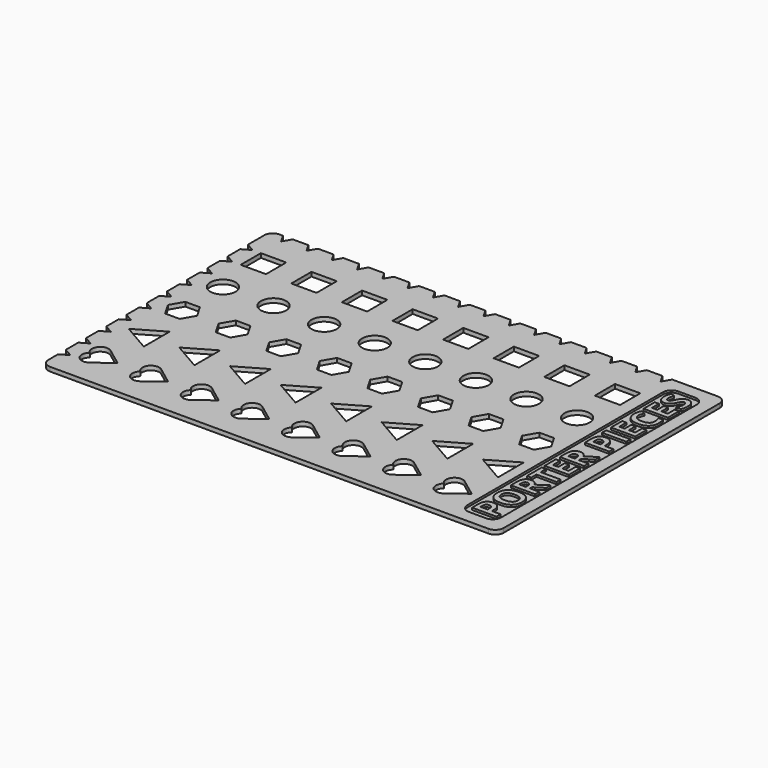
from build123d import *

# Parameters (mm, degrees)
F0_W          = 85.725
F0_H          = 53.975
F1_DEPTH      = 0.79375
F2_R          = 1.5875
F3_W          = 4.7625
F3_H          = 4.7625
F4_DEPTH      = 25.4
F6_DEPTH      = 25.4
F8_DEPTH      = 25.4
F9_R          = 2.38125
F10_DEPTH     = 25.4
F12_DEPTH     = 25.4
F14_DEPTH     = 25.4
F16_DEPTH     = 25.4
F18_DEPTH     = 25.4
F19_W         = 6.35
F19_H         = 49.2125
F20_DEPTH     = 0.396875
F21_R         = 1.5875
F22_TEXT_SIZE = 6.4051106395
F23_DEPTH     = 0.396875
F25_DEPTH     = 25.4
F27_DEPTH     = 25.4


# Not quite as in the source:
# - a feature names something its author has since deleted; it is built from what else it names
# - Text() gives the source's letters only with a copy of the font that has no kerning and outlines rounded to 1/6400 em; it was checked with that copy


with BuildPart() as f1:
    # F0 (on Top) → F1 (new body)
    with BuildSketch(Plane.XY):
        Rectangle(F0_W, F0_H)
    extrude(amount=F1_DEPTH)

    # F2
    f2_edges = [f1.edges().sort_by_distance(p)[0] for p in [
        (42.8625, 26.9875, 0.396875),
        (-42.8625, 26.9875, 0.396875),
        (-42.8625, -26.9875, 0.396875),
        (42.8625, -26.9875, 0.396875),
    ]]
    fillet(f2_edges, radius=F2_R)

    # F3 (on face) → F4 (cut)
    with BuildSketch(Plane.XY.offset(0.79375)):
        with Locations((-37.30625, 18.25625)):
            Rectangle(F3_W, F3_H)
        with Locations((-27.78125, 18.25625)):
            Rectangle(F3_W, F3_H)
        with Locations((-18.25625, 18.25625)):
            Rectangle(F3_W, F3_H)
        with Locations((-8.73125, 18.25625)):
            Rectangle(F3_W, F3_H)
        with Locations((0.79375, 18.25625)):
            Rectangle(F3_W, F3_H)
        with Locations((10.31875, 18.25625)):
            Rectangle(F3_W, F3_H)
        with Locations((19.84375, 18.25625)):
            Rectangle(F3_W, F3_H)
        with Locations((29.36875, 18.25625)):
            Rectangle(F3_W, F3_H)
    extrude(amount=-F4_DEPTH, mode=Mode.SUBTRACT)

    # F5 (on face) → F6 (cut)
    with BuildSketch(Plane.XY.offset(0.79375)):
        Polygon((-34.0084564477, 26.9875), (-35.8415435523, 26.9875), (-34.925, 25.4), align=None)
        Polygon((-29.2459564477, 26.9875), (-31.0790435523, 26.9875), (-30.1625, 25.4), align=None)
        Polygon((-24.4834564477, 26.9875), (-26.3165435523, 26.9875), (-25.4, 25.4), align=None)
        Polygon((-19.7209564477, 26.9875), (-21.5540435523, 26.9875), (-20.6375, 25.4), align=None)
        Polygon((-14.9584564477, 26.9875), (-16.7915435523, 26.9875), (-15.875, 25.4), align=None)
        Polygon((-10.1959564477, 26.9875), (-12.0290435523, 26.9875), (-11.1125, 25.4), align=None)
        Polygon((-5.4334564477, 26.9875), (-7.2665435523, 26.9875), (-6.35, 25.4), align=None)
        Polygon((-0.6709564477, 26.9875), (-2.5040435523, 26.9875), (-1.5875, 25.4), align=None)
        Polygon((8.8540435523, 26.9875), (7.0209564477, 26.9875), (7.9375, 25.4), align=None)
        Polygon((4.0915435523, 26.9875), (2.2584564477, 26.9875), (3.175, 25.4), align=None)
        Polygon((12.7, 25.4), (13.6165435523, 26.9875), (11.7834564477, 26.9875), align=None)
        Polygon((17.4625, 25.4), (18.3790435523, 26.9875), (16.5459564477, 26.9875), align=None)
        Polygon((31.75, 25.4), (32.6665435523, 26.9875), (30.8334564477, 26.9875), align=None)
        Polygon((26.9875, 25.4), (27.9040435523, 26.9875), (26.0709564477, 26.9875), align=None)
        Polygon((22.225, 25.4), (23.1415435523, 26.9875), (21.3084564477, 26.9875), align=None)
    extrude(amount=-F6_DEPTH, mode=Mode.SUBTRACT)

    # F7 (on face) → F8 (cut)
    with BuildSketch(Plane.XY.offset(0.79375)):
        Polygon((-38.7709564477, 26.9875), (-40.6040435523, 26.9875), (-39.6875, 25.4), align=None)
    extrude(amount=-F8_DEPTH, mode=Mode.SUBTRACT)

    # F9 (on face) → F10 (cut)
    with BuildSketch(Plane.XY.offset(0.79375)):
        with Locations((-37.30625, 8.73125)):
            Circle(F9_R)
        with Locations((-27.78125, 8.73125)):
            Circle(F9_R)
        with Locations((-18.25625, 8.73125)):
            Circle(F9_R)
        with Locations((-8.73125, 8.73125)):
            Circle(F9_R)
        with Locations((0.79375, 8.73125)):
            Circle(F9_R)
        with Locations((10.31875, 8.73125)):
            Circle(F9_R)
        with Locations((19.84375, 8.73125)):
            Circle(F9_R)
        with Locations((29.36875, 8.73125)):
            Circle(F9_R)
    extrude(amount=-F10_DEPTH, mode=Mode.SUBTRACT)

    # F11 (on face) → F12 (cut)
    with BuildSketch(Plane.XY.offset(0.79375)):
        Polygon((-35.9314346715, 1.5875), (-38.6810653285, 1.5875), (-40.055880657, -0.79375), (-38.6810653285, -3.175), (-35.9314346715, -3.175), (-34.556619343, -0.79375), align=None)
        Polygon((-26.4064346715, 1.5875), (-29.1560653285, 1.5875), (-30.530880657, -0.79375), (-29.1560653285, -3.175), (-26.4064346715, -3.175), (-25.031619343, -0.79375), align=None)
        Polygon((-16.8814346715, 1.5875), (-19.6310653285, 1.5875), (-21.005880657, -0.79375), (-19.6310653285, -3.175), (-16.8814346715, -3.175), (-15.506619343, -0.79375), align=None)
        Polygon((-7.3564346715, 1.5875), (-10.1060653285, 1.5875), (-11.480880657, -0.79375), (-10.1060653285, -3.175), (-7.3564346715, -3.175), (-5.981619343, -0.79375), align=None)
        Polygon((2.1685653285, 1.5875), (-0.5810653285, 1.5875), (-1.955880657, -0.79375), (-0.5810653285, -3.175), (2.1685653285, -3.175), (3.543380657, -0.79375), align=None)
        Polygon((11.6935653285, 1.5875), (8.9439346715, 1.5875), (7.569119343, -0.79375), (8.9439346715, -3.175), (11.6935653285, -3.175), (13.068380657, -0.79375), align=None)
        Polygon((21.2185653285, 1.5875), (18.4689346715, 1.5875), (17.094119343, -0.79375), (18.4689346715, -3.175), (21.2185653285, -3.175), (22.593380657, -0.79375), align=None)
        Polygon((30.7435653285, 1.5875), (27.9939346715, 1.5875), (26.619119343, -0.79375), (27.9939346715, -3.175), (30.7435653285, -3.175), (32.118380657, -0.79375), align=None)
    extrude(amount=-F12_DEPTH, mode=Mode.SUBTRACT)

    # F13 (on face) → F14 (cut)
    with BuildSketch(Plane.XY.offset(0.79375)):
        Polygon((-34.925, -12.7), (-34.925, -7.9375), (-39.0494459855, -10.31875), align=None)
        Polygon((-25.4, -7.9375), (-29.5244459855, -10.31875), (-25.4, -12.7), align=None)
        Polygon((-15.875, -7.9375), (-19.9994459855, -10.31875), (-15.875, -12.7), align=None)
        Polygon((-6.35, -7.9375), (-10.4744459855, -10.31875), (-6.35, -12.7), align=None)
        Polygon((3.175, -7.9375), (-0.9494459855, -10.31875), (3.175, -12.7), align=None)
        Polygon((12.7, -7.9375), (8.5755540145, -10.31875), (12.7, -12.7), align=None)
        Polygon((22.225, -7.9375), (18.1005540145, -10.31875), (22.225, -12.7), align=None)
        Polygon((31.75, -7.9375), (27.6255540145, -10.31875), (31.75, -12.7), align=None)
    extrude(amount=-F14_DEPTH, mode=Mode.SUBTRACT)

    # F15 (on face) → F16 (cut)
    with BuildSketch(Plane.XY.offset(0.79375)):
        with BuildLine():
            ThreePointArc((-37.7825, -17.700625), (-39.6264010517, -18.2766163161), (-38.496875, -19.84375))
            ThreePointArc((-38.496875, -19.84375), (-39.6264010517, -21.4108836839), (-37.7825, -21.986875))
            Line((-37.7825, -21.986875), (-34.925, -19.84375))
            Line((-34.925, -19.84375), (-37.7825, -17.700625))
        make_face()
        with BuildLine():
            ThreePointArc((-28.2575, -17.700625), (-30.1014010517, -18.2766163161), (-28.971875, -19.84375))
            ThreePointArc((-28.971875, -19.84375), (-30.1014010517, -21.4108836839), (-28.2575, -21.986875))
            Line((-28.2575, -21.986875), (-25.4, -19.84375))
            Line((-25.4, -19.84375), (-28.2575, -17.700625))
        make_face()
        with BuildLine():
            ThreePointArc((-18.7325, -17.700625), (-20.5764010517, -18.2766163161), (-19.446875, -19.84375))
            ThreePointArc((-19.446875, -19.84375), (-20.5764010517, -21.4108836839), (-18.7325, -21.986875))
            Line((-18.7325, -21.986875), (-15.875, -19.84375))
            Line((-15.875, -19.84375), (-18.7325, -17.700625))
        make_face()
        with BuildLine():
            ThreePointArc((-9.2075, -17.700625), (-11.0514010517, -18.2766163161), (-9.921875, -19.84375))
            ThreePointArc((-9.921875, -19.84375), (-11.0514010517, -21.4108836839), (-9.2075, -21.986875))
            Line((-9.2075, -21.986875), (-6.35, -19.84375))
            Line((-6.35, -19.84375), (-9.2075, -17.700625))
        make_face()
        with BuildLine():
            ThreePointArc((0.3175, -17.700625), (-1.5264010517, -18.2766163161), (-0.396875, -19.84375))
            ThreePointArc((-0.396875, -19.84375), (-1.5264010517, -21.4108836839), (0.3175, -21.986875))
            Line((0.3175, -21.986875), (3.175, -19.84375))
            Line((3.175, -19.84375), (0.3175, -17.700625))
        make_face()
        with BuildLine():
            ThreePointArc((9.8425, -17.700625), (7.9985989483, -18.2766163161), (9.128125, -19.84375))
            ThreePointArc((9.128125, -19.84375), (7.9985989483, -21.4108836839), (9.8425, -21.986875))
            Line((9.8425, -21.986875), (12.7, -19.84375))
            Line((12.7, -19.84375), (9.8425, -17.700625))
        make_face()
        with BuildLine():
            ThreePointArc((19.3675, -17.700625), (17.5235989483, -18.2766163161), (18.653125, -19.84375))
            ThreePointArc((18.653125, -19.84375), (17.5235989483, -21.4108836839), (19.3675, -21.986875))
            Line((19.3675, -21.986875), (22.225, -19.84375))
            Line((22.225, -19.84375), (19.3675, -17.700625))
        make_face()
        with BuildLine():
            ThreePointArc((28.8925, -17.700625), (27.0485989483, -18.2766163161), (28.178125, -19.84375))
            ThreePointArc((28.178125, -19.84375), (27.0485989483, -21.4108836839), (28.8925, -21.986875))
            Line((28.8925, -21.986875), (31.75, -19.84375))
            Line((31.75, -19.84375), (28.8925, -17.700625))
        make_face()
    extrude(amount=-F16_DEPTH, mode=Mode.SUBTRACT)

    # F17 (on face) → F18 (cut)
    with BuildSketch(Plane(origin=(0, 0, 0), x_dir=(1, 0, 0), z_dir=(0, 0, -1))):
        Polygon((-42.8625, -19.7209564477), (-42.8625, -21.5540435523), (-41.275, -20.6375), align=None)
        Polygon((-42.8625, -14.9584564477), (-42.8625, -16.7915435523), (-41.275, -15.875), align=None)
        Polygon((-42.8625, -10.1959564477), (-42.8625, -12.0290435523), (-41.275, -11.1125), align=None)
        Polygon((-42.8625, -5.4334564477), (-42.8625, -7.2665435523), (-41.275, -6.35), align=None)
        Polygon((-42.8625, -0.6709564477), (-42.8625, -2.5040435523), (-41.275, -1.5875), align=None)
        Polygon((-42.8625, 4.0915435523), (-42.8625, 2.2584564477), (-41.275, 3.175), align=None)
        Polygon((-42.8625, 8.8540435523), (-42.8625, 7.0209564477), (-41.275, 7.9375), align=None)
        Polygon((-42.8625, 13.6165435523), (-42.8625, 11.7834564477), (-41.275, 12.7), align=None)
        Polygon((-42.8625, 18.3790435523), (-42.8625, 16.5459564477), (-41.275, 17.4625), align=None)
        Polygon((-42.8625, 23.1415435523), (-42.8625, 21.3084564477), (-41.275, 22.225), align=None)
    extrude(amount=-F18_DEPTH, mode=Mode.SUBTRACT)

    # F19 (on face) → F20 (cut)
    with BuildSketch(Plane.XY.offset(0.79375)):
        with Locations((37.30625, 0)):
            Rectangle(F19_W, F19_H)
    extrude(amount=-F20_DEPTH, mode=Mode.SUBTRACT)

    # F21
    f21_edges = [f1.edges().sort_by_distance(p)[0] for p in [
        (34.13125, -24.60625, 0.595313),
        (40.48125, -24.60625, 0.595313),
        (40.48125, 24.60625, 0.595313),
        (34.13125, 24.60625, 0.595313),
    ]]
    fillet(f21_edges, radius=F21_R)

    # F22 (on face) → F23 (join)
    with BuildSketch(Plane.XY.offset(0.396875)):
        with Locations(Location((39.7566241945, -23.8125), (0, 0, 90))):
            Text('PORTER PIECES', F22_TEXT_SIZE, font='Open Sans', font_style=FontStyle.BOLD, text_align=(TextAlign.LEFT, TextAlign.BOTTOM))
    extrude(amount=F23_DEPTH)

    # F24 (on face) → F25 (cut)
    with BuildSketch(Plane.XY.offset(0.79375)):
        Polygon((-39.8114459855, -10.31875), (-34.544, -13.3599113577), (-34.544, -7.2775886423), align=None)
        Polygon((-34.925, -7.9375), (-34.925, -12.7), (-39.0494459855, -10.31875), align=None, mode=Mode.SUBTRACT)
        Polygon((-25.019, -13.3599113577), (-25.019, -7.2775886423), (-30.2864459855, -10.31875), align=None)
        Polygon((-25.4, -12.7), (-29.5244459855, -10.31875), (-25.4, -7.9375), align=None, mode=Mode.SUBTRACT)
        Polygon((-15.494, -13.3599113577), (-15.494, -7.2775886423), (-20.7614459855, -10.31875), align=None)
        Polygon((-15.875, -12.7), (-19.9994459855, -10.31875), (-15.875, -7.9375), align=None, mode=Mode.SUBTRACT)
        Polygon((-5.969, -13.3599113577), (-5.969, -7.2775886423), (-11.2364459855, -10.31875), align=None)
        Polygon((-6.35, -12.7), (-10.4744459855, -10.31875), (-6.35, -7.9375), align=None, mode=Mode.SUBTRACT)
        Polygon((3.556, -13.3599113577), (3.556, -7.2775886423), (-1.7114459855, -10.31875), align=None)
        Polygon((3.175, -12.7), (-0.9494459855, -10.31875), (3.175, -7.9375), align=None, mode=Mode.SUBTRACT)
        Polygon((13.081, -13.3599113577), (13.081, -7.2775886423), (7.8135540145, -10.31875), align=None)
        Polygon((12.7, -12.7), (8.5755540145, -10.31875), (12.7, -7.9375), align=None, mode=Mode.SUBTRACT)
        Polygon((22.606, -13.3599113577), (22.606, -7.2775886423), (17.3385540145, -10.31875), align=None)
        Polygon((22.225, -12.7), (18.1005540145, -10.31875), (22.225, -7.9375), align=None, mode=Mode.SUBTRACT)
        Polygon((32.131, -13.3599113577), (32.131, -7.2775886423), (26.8635540145, -10.31875), align=None)
        Polygon((31.75, -12.7), (27.6255540145, -10.31875), (31.75, -7.9375), align=None, mode=Mode.SUBTRACT)
    extrude(amount=-F25_DEPTH, mode=Mode.SUBTRACT)

    # F26 (on face) → F27 (cut)
    with BuildSketch(Plane.XY.offset(0.79375)):
        with BuildLine():
            Line((-37.5539, -22.291675), (-34.29, -19.84375))
            Line((-34.29, -19.84375), (-37.5539, -17.395825))
            ThreePointArc((-37.5539, -17.395825), (-39.721539141, -17.6681362272), (-39.5227488958, -19.84375))
            ThreePointArc((-39.5227488958, -19.84375), (-39.721539141, -22.0193637728), (-37.5539, -22.291675))
        make_face()
        with BuildLine():
            ThreePointArc((-37.7825, -21.986875), (-39.6264010517, -21.4108836839), (-38.496875, -19.84375))
            ThreePointArc((-38.496875, -19.84375), (-39.6264010517, -18.2766163161), (-37.7825, -17.700625))
            Line((-37.7825, -17.700625), (-34.925, -19.84375))
            Line((-34.925, -19.84375), (-37.7825, -21.986875))
        make_face(mode=Mode.SUBTRACT)
        with BuildLine():
            Line((-28.0289, -22.291675), (-24.765, -19.84375))
            Line((-24.765, -19.84375), (-28.0289, -17.395825))
            ThreePointArc((-28.0289, -17.395825), (-30.196539141, -17.6681362272), (-29.9977488958, -19.84375))
            ThreePointArc((-29.9977488958, -19.84375), (-30.196539141, -22.0193637728), (-28.0289, -22.291675))
        make_face()
        with BuildLine():
            ThreePointArc((-28.971875, -19.84375), (-30.1014010517, -18.2766163161), (-28.2575, -17.700625))
            Line((-28.2575, -17.700625), (-25.4, -19.84375))
            Line((-25.4, -19.84375), (-28.2575, -21.986875))
            ThreePointArc((-28.2575, -21.986875), (-30.1014010517, -21.4108836839), (-28.971875, -19.84375))
        make_face(mode=Mode.SUBTRACT)
        with BuildLine():
            Line((-18.5039, -22.291675), (-15.24, -19.84375))
            Line((-15.24, -19.84375), (-18.5039, -17.395825))
            ThreePointArc((-18.5039, -17.395825), (-20.671539141, -17.6681362272), (-20.4727488958, -19.84375))
            ThreePointArc((-20.4727488958, -19.84375), (-20.671539141, -22.0193637728), (-18.5039, -22.291675))
        make_face()
        with BuildLine():
            Line((-18.7325, -17.700625), (-15.875, -19.84375))
            Line((-15.875, -19.84375), (-18.7325, -21.986875))
            ThreePointArc((-18.7325, -21.986875), (-20.5764010517, -21.4108836839), (-19.446875, -19.84375))
            ThreePointArc((-19.446875, -19.84375), (-20.5764010517, -18.2766163161), (-18.7325, -17.700625))
        make_face(mode=Mode.SUBTRACT)
        with BuildLine():
            Line((-8.9789, -22.291675), (-5.715, -19.84375))
            Line((-5.715, -19.84375), (-8.9789, -17.395825))
            ThreePointArc((-8.9789, -17.395825), (-11.146539141, -17.6681362272), (-10.9477488958, -19.84375))
            ThreePointArc((-10.9477488958, -19.84375), (-11.146539141, -22.0193637728), (-8.9789, -22.291675))
        make_face()
        with BuildLine():
            ThreePointArc((-9.921875, -19.84375), (-11.0514010517, -18.2766163161), (-9.2075, -17.700625))
            Line((-9.2075, -17.700625), (-6.35, -19.84375))
            Line((-6.35, -19.84375), (-9.2075, -21.986875))
            ThreePointArc((-9.2075, -21.986875), (-11.0514010517, -21.4108836839), (-9.921875, -19.84375))
        make_face(mode=Mode.SUBTRACT)
        with BuildLine():
            Line((0.5461, -22.291675), (3.81, -19.84375))
            Line((3.81, -19.84375), (0.5461, -17.395825))
            ThreePointArc((0.5461, -17.395825), (-1.621539141, -17.6681362272), (-1.4227488958, -19.84375))
            ThreePointArc((-1.4227488958, -19.84375), (-1.621539141, -22.0193637728), (0.5461, -22.291675))
        make_face()
        with BuildLine():
            Line((0.3175, -17.700625), (3.175, -19.84375))
            Line((3.175, -19.84375), (0.3175, -21.986875))
            ThreePointArc((0.3175, -21.986875), (-1.5264010517, -21.4108836839), (-0.396875, -19.84375))
            ThreePointArc((-0.396875, -19.84375), (-1.5264010517, -18.2766163161), (0.3175, -17.700625))
        make_face(mode=Mode.SUBTRACT)
        with BuildLine():
            Line((29.1211, -22.291675), (32.385, -19.84375))
            Line((32.385, -19.84375), (29.1211, -17.395825))
            ThreePointArc((29.1211, -17.395825), (26.953460859, -17.6681362272), (27.1522511042, -19.84375))
            ThreePointArc((27.1522511042, -19.84375), (26.953460859, -22.0193637728), (29.1211, -22.291675))
        make_face()
        with BuildLine():
            ThreePointArc((28.8925, -21.986875), (27.0485989483, -21.4108836839), (28.178125, -19.84375))
            ThreePointArc((28.178125, -19.84375), (27.0485989483, -18.2766163161), (28.8925, -17.700625))
            Line((28.8925, -17.700625), (31.75, -19.84375))
            Line((31.75, -19.84375), (28.8925, -21.986875))
        make_face(mode=Mode.SUBTRACT)
        with BuildLine():
            Line((19.5961, -22.291675), (22.86, -19.84375))
            Line((22.86, -19.84375), (19.5961, -17.395825))
            ThreePointArc((19.5961, -17.395825), (17.428460859, -17.6681362272), (17.6272511042, -19.84375))
            ThreePointArc((17.6272511042, -19.84375), (17.428460859, -22.0193637728), (19.5961, -22.291675))
        make_face()
        with BuildLine():
            Line((19.3675, -17.700625), (22.225, -19.84375))
            Line((22.225, -19.84375), (19.3675, -21.986875))
            ThreePointArc((19.3675, -21.986875), (17.5235989483, -21.4108836839), (18.653125, -19.84375))
            ThreePointArc((18.653125, -19.84375), (17.5235989483, -18.2766163161), (19.3675, -17.700625))
        make_face(mode=Mode.SUBTRACT)
        with BuildLine():
            Line((10.0711, -22.291675), (13.335, -19.84375))
            Line((13.335, -19.84375), (10.0711, -17.395825))
            ThreePointArc((10.0711, -17.395825), (7.903460859, -17.6681362272), (8.1022511042, -19.84375))
            ThreePointArc((8.1022511042, -19.84375), (7.903460859, -22.0193637728), (10.0711, -22.291675))
        make_face()
        with BuildLine():
            ThreePointArc((9.128125, -19.84375), (7.9985989483, -18.2766163161), (9.8425, -17.700625))
            Line((9.8425, -17.700625), (12.7, -19.84375))
            Line((12.7, -19.84375), (9.8425, -21.986875))
            ThreePointArc((9.8425, -21.986875), (7.9985989483, -21.4108836839), (9.128125, -19.84375))
        make_face(mode=Mode.SUBTRACT)
    extrude(amount=-F27_DEPTH, mode=Mode.SUBTRACT)


solid = f1.part
